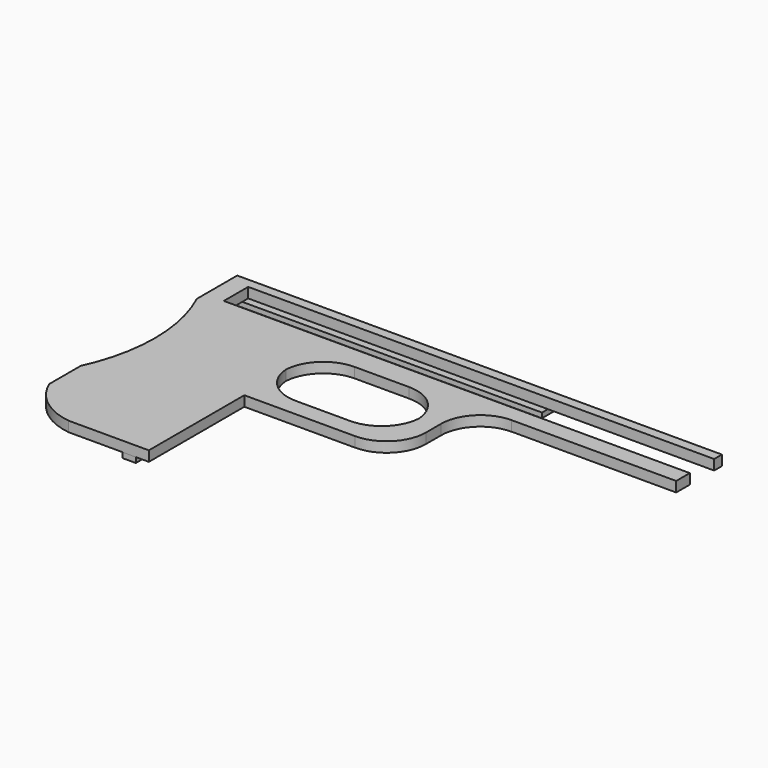
from build123d import *

# Parameters (mm, degrees)
F0_W         = 142.9656147957
F0_H         = 80.8112323284
F1_DEPTH     = 3
F2_W         = 137.4550536275
F2_H         = 8.9848991483
F2_W_2       = 60.0944850594
F2_H_2       = 18.4983238578
F3_DEPTH     = 52.3
F4_W         = 39.2408655025
F4_H         = 21.6958951205
F5_DEPTH     = 25
F6_W         = 3.3521875739
F6_H         = 44.7733802721
F6_W_2       = 40.9712046385
F7_DEPTH     = 25
F8_W         = 102.604271844
F8_H         = 18.422623165
F9_DEPTH     = 25
F10_T1_DEPTH = 3
F10_T3_DEPTH = 60.941125497
F12_DEPTH    = 25
F14_DEPTH    = 25
F16_DEPTH    = 25
F17_W        = 93.9226467162
F17_H        = 5.0384774804
F18_DEPTH    = 1.4789979905
F19_W        = 52.2845312953
F19_H        = 2.1970570087
F20_DEPTH    = 0.8268505335
F21_DEPTH    = 0.7327459753
F22_W        = 3.9923638105
F22_H        = 1.5595965087
F23_DEPTH    = 65.8853985369
F24_W        = 7.4088871479
F24_H        = 1.9754432142
F25_DEPTH    = 1.11994287


# Not quite as in the source:
# - a fillet or chamfer that OpenCascade refuses, or shapes differently, is made with other operations: its cross-section is extruded or revolved along the edge and cut away or added


with BuildPart() as f1:
    # F0 (on Top) → F1 (new body)
    with BuildSketch(Plane.XY):
        Rectangle(F0_W, F0_H)
    extrude(amount=F1_DEPTH)

    # F2 (on face) → F3 (cut)
    with BuildSketch(Plane.XY.offset(3)):
        with Locations((2.7552805841, 33.0591509119)):
            Rectangle(F2_W, F2_H)
        with Locations((41.4355648682, 14.2965670675)):
            Rectangle(F2_W_2, F2_H_2)
    extrude(amount=-F3_DEPTH, mode=Mode.SUBTRACT)

    # F4 (on face) → F5 (cut)
    with BuildSketch(Plane.XY.offset(3)):
        with Locations((-13.8379565906, 10.8479475603)):
            Rectangle(F4_W, F4_H)
    extrude(amount=-F5_DEPTH, mode=Mode.SUBTRACT)

    # F6 (on face) → F7 (cut)
    with BuildSketch(Plane.XY.offset(3)):
        Polygon((98.6725464463, 0), (13.7504395097, 0), (13.7504395097, -5.2010240033), (17.1026270837, -5.2010240033), (17.1026270837, -49.9744042754), (13.7504395097, -49.9744042754), (13.7504395097, -55.2418604493), (98.6725464463, -55.2418604493), align=None)
        with Locations((15.4265332967, -27.5877141394)):
            Rectangle(F6_W, F6_H)
        with Locations((-6.7351628095, -27.5877141394)):
            Rectangle(F6_W_2, F6_H)
    extrude(amount=-F7_DEPTH, mode=Mode.SUBTRACT)

    # F8 (on face) → F9 (cut)
    with BuildSketch(Plane.XY.offset(3)):
        with Locations((62.6904582605, -4.1639064439)):
            Rectangle(F8_W, F8_H)
    extrude(amount=-F9_DEPTH, mode=Mode.SUBTRACT)

    # F10: fillet of radius 11.5882250994 on 7 edges, made by hand

    # F10_s2 → F10_t1 (join)
    with BuildSketch(Plane.XY):
        with BuildLine():
            ThreePointArc((22.9765474379, 23.5457289964), (14.7824348882, 20.1516164467), (11.3883223385, 11.957503897))
            Line((11.3883223385, 11.957503897), (11.3883223385, 23.5457289964))
            Line((11.3883223385, 23.5457289964), (22.9765474379, 23.5457289964))
        make_face()
        with BuildLine():
            ThreePointArc((-15.6325400293, -5.2010240033), (-23.826652579, -8.595136553), (-27.2207651287, -16.7892491027))
            Line((-27.2207651287, -16.7892491027), (-27.2207651287, -5.2010240033))
            Line((-27.2207651287, -5.2010240033), (-15.6325400293, -5.2010240033))
        make_face()
        with BuildLine():
            ThreePointArc((-33.4583893418, 10.1076700211), (-30.0642767921, 18.3017825708), (-21.8701642424, 21.6958951205))
            Line((-21.8701642424, 21.6958951205), (-33.4583893418, 21.6958951205))
            Line((-33.4583893418, 21.6958951205), (-33.4583893418, 10.1076700211))
        make_face()
        with BuildLine():
            ThreePointArc((-5.8057489387, 0), (2.388363611, 3.3941125497), (5.7824761607, 11.5882250994))
            Line((5.7824761607, 11.5882250994), (5.7824761607, 0))
            Line((5.7824761607, 0), (-5.8057489387, 0))
        make_face()
        with BuildLine():
            ThreePointArc((-33.4583893418, 11.5882250994), (-30.0642767921, 3.3941125497), (-21.8701642424, 0))
            Line((-21.8701642424, 0), (-33.4583893418, 0))
            Line((-33.4583893418, 0), (-33.4583893418, 11.5882250994))
        make_face()
        with BuildLine():
            ThreePointArc((5.7824761607, 10.1076700211), (2.388363611, 18.3017825708), (-5.8057489387, 21.6958951205))
            Line((-5.8057489387, 21.6958951205), (5.7824761607, 21.6958951205))
            Line((5.7824761607, 21.6958951205), (5.7824761607, 10.1076700211))
        make_face()
    extrude(amount=F10_T1_DEPTH)

    # F10_s4 → F10_t3 (cut)
    with BuildSketch(Plane.XY.offset(-28.9705627485)):
        with BuildLine():
            ThreePointArc((-0.1999027609, -5.2010240033), (7.9942097888, -1.8069114536), (11.3883223385, 6.3872010961))
            Line((11.3883223385, 6.3872010961), (11.3883223385, -5.2010240033))
            Line((11.3883223385, -5.2010240033), (-0.1999027609, -5.2010240033))
        make_face()
    extrude(amount=F10_T3_DEPTH, mode=Mode.SUBTRACT)

    # F11 (on face) → F12 (cut)
    with BuildSketch(Plane.XY.offset(3)):
        with BuildLine():
            Line((-71.4828073978, 25.5012605339), (-71.4828073978, -17.3091441393))
            ThreePointArc((-71.4828073978, -17.3091441393), (-66.7668008007, 4.0960581973), (-71.4828073978, 25.5012605339))
        make_face()
    extrude(amount=-F12_DEPTH, mode=Mode.SUBTRACT)

    # F13 (on face) → F14 (cut)
    with BuildSketch(Plane.XY.offset(3)):
        with BuildLine():
            ThreePointArc((-21.3245461018, -6.6952891353), (-30.1185964093, -13.4662376926), (-27.2207651287, -24.1799503565))
            Line((-27.2207651287, -24.1799503565), (-27.2207651287, -16.7892491027))
            ThreePointArc((-27.2207651287, -16.7892491027), (-25.6387183355, -10.944306275), (-21.3245461018, -6.6952891353))
        make_face()
        with BuildLine():
            ThreePointArc((-27.2207651287, -32.8327932205), (-29.4171017882, -37.101902666), (-32.9005867243, -40.4056161642))
            Line((-32.9005867243, -40.4056161642), (-27.2207651287, -40.4056161642))
            Line((-27.2207651287, -40.4056161642), (-27.2207651287, -32.8327932205))
        make_face()
        with BuildLine():
            ThreePointArc((-56.574376872, -40.4056161642), (-65.5880780241, -36.6447482344), (-71.4828073978, -28.8573801517))
            Line((-71.4828073978, -28.8573801517), (-71.4828073978, -40.4056161642))
            Line((-71.4828073978, -40.4056161642), (-56.574376872, -40.4056161642))
        make_face()
    extrude(amount=-F14_DEPTH, mode=Mode.SUBTRACT)

    # F15 (on face) → F16 (cut)
    with BuildSketch(Plane.XY.offset(3)):
        with BuildLine():
            Line((-32.9005867243, -5.2010240033), (-32.9005867243, -40.4056161642))
            ThreePointArc((-32.9005867243, -40.4056161642), (-29.4171017882, -37.101902666), (-27.2207651287, -32.8327932205))
            Line((-27.2207651287, -32.8327932205), (-27.2207651287, -24.1799503565))
            ThreePointArc((-27.2207651287, -24.1799503565), (-30.1185964093, -13.4662376926), (-21.3245461018, -6.6952891353))
            ThreePointArc((-21.3245461018, -6.6952891353), (-18.5749778542, -5.5808138595), (-15.6325400293, -5.2010240033))
            Line((-15.6325400293, -5.2010240033), (-32.9005867243, -5.2010240033))
        make_face()
    extrude(amount=-F16_DEPTH, mode=Mode.SUBTRACT)

    # F17 (on face) → F18 (join)
    with BuildSketch(Plane(origin=(0, 0, 0), x_dir=(1, 0, 0), z_dir=(0, 0, -1))):
        with Locations((-24.5214840397, -37.886377424)):
            Rectangle(F17_W, F17_H)
    extrude(amount=F18_DEPTH)

    # F19 (on face) → F20 (join)
    with BuildSketch(Plane(origin=(0, 0, 0), x_dir=(1, 0, 0), z_dir=(0, 0, -1))):
        with Locations((-39.829980582, -29.6652298421)):
            Rectangle(F19_W, F19_H)
        Polygon((-71.4828073978, -30.7637583464), (-65.9722462296, -30.7637583464), (-65.9722462296, -28.5667013377), (-13.6877149343, -28.5667013377), (-13.6877149343, -25.5012605339), (-71.4828073978, -25.5012605339), align=None)
    extrude(amount=F20_DEPTH)

    # F21 (add): a face of the model
    f21_faces = [f1.faces().sort_by_distance(p)[0] for p in [
        (-42.5852611661, 28.1325094402, -0.8268505335),
    ]]
    extrude(f21_faces, amount=F21_DEPTH)

    # F22 (on face) → F23 (join)
    with BuildSketch(Plane.XZ.offset(-25.5012605339)):
        with Locations((-38.7431830168, -0.7797982544)):
            Rectangle(F22_W, F22_H)
    extrude(amount=F23_DEPTH)

    # F24 (on face) → F25 (join)
    with BuildSketch(Plane(origin=(0, 0, -1.5595965087), x_dir=(1, 0, 0), z_dir=(0, 0, -1))):
        with Locations((-17.3921585083, -30.787916854)):
            Rectangle(F24_W, F24_H)
    extrude(amount=F25_DEPTH)


solid = f1.part
